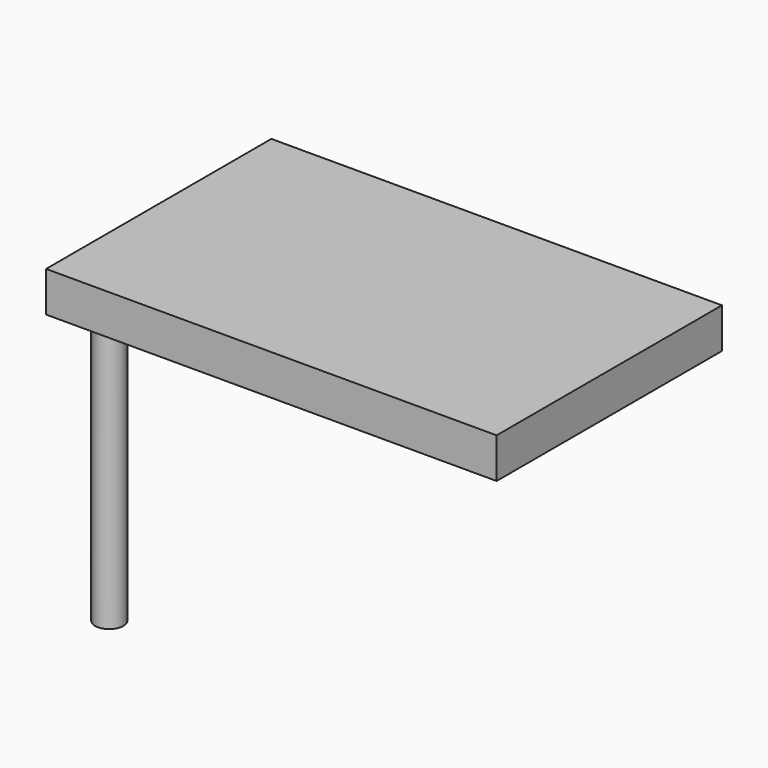
from build123d import *

# Parameters (mm, degrees)
F0_W     = 284.48
F0_H     = 177.8
F1_DEPTH = 25.4
F2_R     = 8.89
F3_DEPTH = 167.64


# Not quite as in the source:
# - the program builds the solid bodies; features that only make, move or delete a surface that nothing else refers to are left out


with BuildPart() as f1:
    # F0 (on Top) → F1 (new body)
    with BuildSketch(Plane.XY):
        with Locations((-8.4218410349, 10.4008839965)):
            Rectangle(F0_W, F0_H)
    extrude(amount=F1_DEPTH)

    # F2 (on face) → F3 (join)
    with BuildSketch(Plane(origin=(0, 0, 0), x_dir=(1, 0, 0), z_dir=(0, 0, -1))):
        with Locations((-123.2527345419, 62.9018843174)):
            Circle(F2_R)
    extrude(amount=F3_DEPTH)


solid = f1.part
